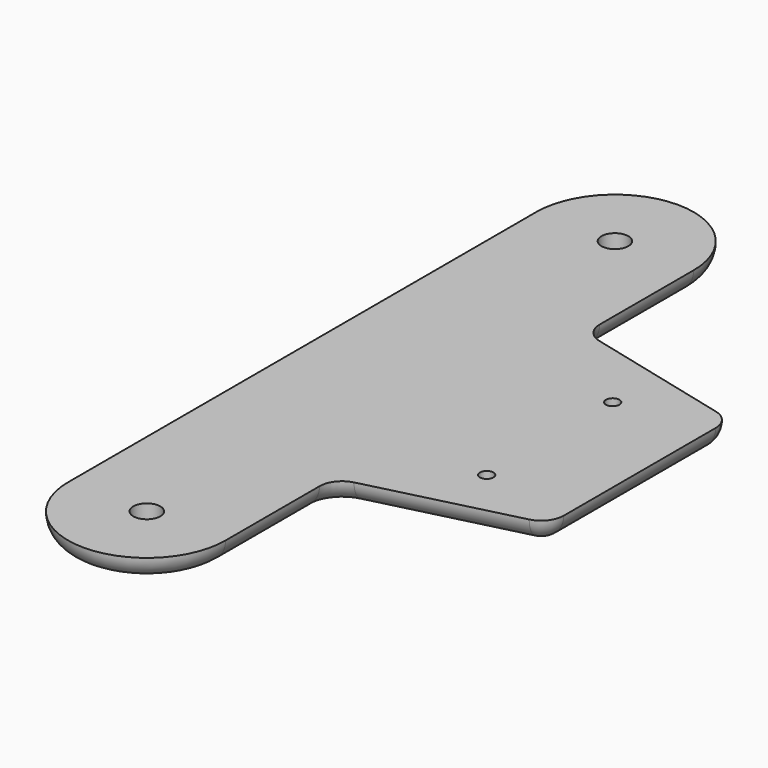
from build123d import *

# Parameters (mm, degrees)
F0_R     = 1.5
F0_R_2   = 3
F1_DEPTH = 5
F2_R     = 4.99999


# Not quite as in the source:
# - a fillet or chamfer is up to 0.001 mm smaller than in the source, because OpenCascade refuses the exact size


with BuildPart() as f1:
    # F0 (on Top) → F1 (new body)
    with BuildSketch(Plane.XY):
        with BuildLine():
            Line((17.5, -65), (17.5, 65))
            ThreePointArc((17.5, 65), (0, 82.5), (-17.5, 65))
            Line((-17.5, 65), (-17.5, 38.903882032))
            ThreePointArc((-17.5, 38.903882032), (-18.5589728099, 35.826820985), (-21.2873218748, 34.0531695313))
            Line((-21.2873218748, 34.0531695313), (-53.7126781252, 25.9468304687))
            ThreePointArc((-53.7126781252, 25.9468304687), (-56.4410271901, 24.173179015), (-57.5, 21.096117968))
            Line((-57.5, 21.096117968), (-57.5, -21.096117968))
            ThreePointArc((-57.5, -21.096117968), (-56.4410271901, -24.173179015), (-53.7126781252, -25.9468304687))
            Line((-53.7126781252, -25.9468304687), (-21.2873218748, -34.0531695313))
            ThreePointArc((-21.2873218748, -34.0531695313), (-18.5589728099, -35.826820985), (-17.5, -38.903882032))
            Line((-17.5, -38.903882032), (-17.5, -65))
            ThreePointArc((-17.5, -65), (0, -82.5), (17.5, -65))
        make_face()
        with Locations((-37.5, -17.5)):
            Circle(F0_R, mode=Mode.SUBTRACT)
        with Locations((0, -65)):
            Circle(F0_R_2, mode=Mode.SUBTRACT)
        with Locations((-37.5, 17.5)):
            Circle(F0_R, mode=Mode.SUBTRACT)
        with Locations((0, 65)):
            Circle(F0_R_2, mode=Mode.SUBTRACT)
    extrude(amount=F1_DEPTH)

    # F2 (radius 5 in the source; OpenCascade refuses exactly that, so slightly less here)
    f2_edges = [f1.edges().sort_by_distance(p)[0] for p in [
        (17.5, 0, 0),
    ]]
    fillet(f2_edges, radius=F2_R)


with BuildPart() as f3_1:
    # F3: instance of F1
    add(f1.part.mirror(Plane.YZ))


solid = f3_1.part
